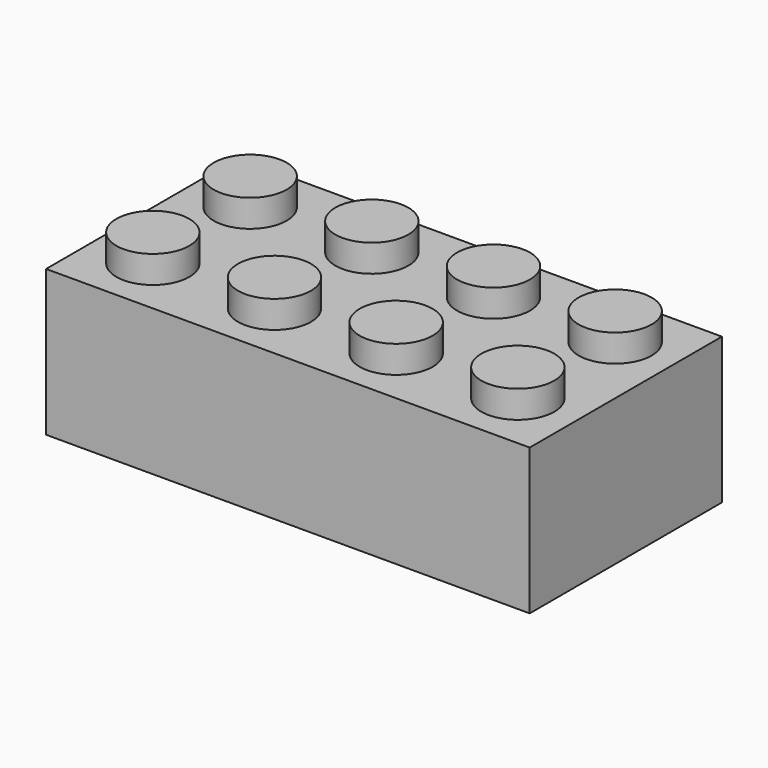
from build123d import *

# Parameters (mm, degrees)
F0_W     = 31.8
F0_H     = 15.8
F1_DEPTH = 9.6
F2_R     = 2.4
F3_DEPTH = 1.8
F4_T     = -1
F5_R     = 3.255
F5_R_2   = 2.4
F6_DEPTH = 8.6


# Not quite as in the source:
# - a pattern or mirror of a feature is missing from the dataset's text; its kind, count and spacing are read off the source's solid


with BuildPart() as f1:
    # F0 (on Top) → F1 (new body)
    with BuildSketch(Plane.XY):
        Rectangle(F0_W, F0_H)
    extrude(amount=F1_DEPTH)

    # F2 (on face) → F3 (join)
    with BuildSketch(Plane.XY.offset(9.6)):
        with Locations((-12, 4)):
            Circle(F2_R)
        with Locations((-4, 4)):
            Circle(F2_R)
        with Locations((4, 4)):
            Circle(F2_R)
        with Locations((12, 4)):
            Circle(F2_R)
    f3 = extrude(amount=F3_DEPTH)

    # F3_copies: F3 across plane
    add(f3.mirror(Plane(origin=(0, 0, 0), x_dir=(0, 0, -1), z_dir=(0, -1, 0))))

    # F4
    f4_openings = [f1.faces().sort_by_distance(p)[0] for p in [
        (0, 0, 0),
    ]]
    offset(amount=F4_T, openings=f4_openings, kind=Kind.INTERSECTION)

    # F5 (on face) → F6 (join, through all)
    with BuildSketch(Plane(origin=(0, 0, 8.6), x_dir=(1, 0, 0), z_dir=(0, 0, -1))):
        with Locations((-8, 0)):
            Circle(F5_R)
        with Locations((-8, 0)):
            Circle(F5_R_2, mode=Mode.SUBTRACT)
        Circle(F5_R)
        Circle(F5_R_2, mode=Mode.SUBTRACT)
        with Locations((8, 0)):
            Circle(F5_R)
        with Locations((8, 0)):
            Circle(F5_R_2, mode=Mode.SUBTRACT)
    extrude(amount=F6_DEPTH)


solid = f1.part
